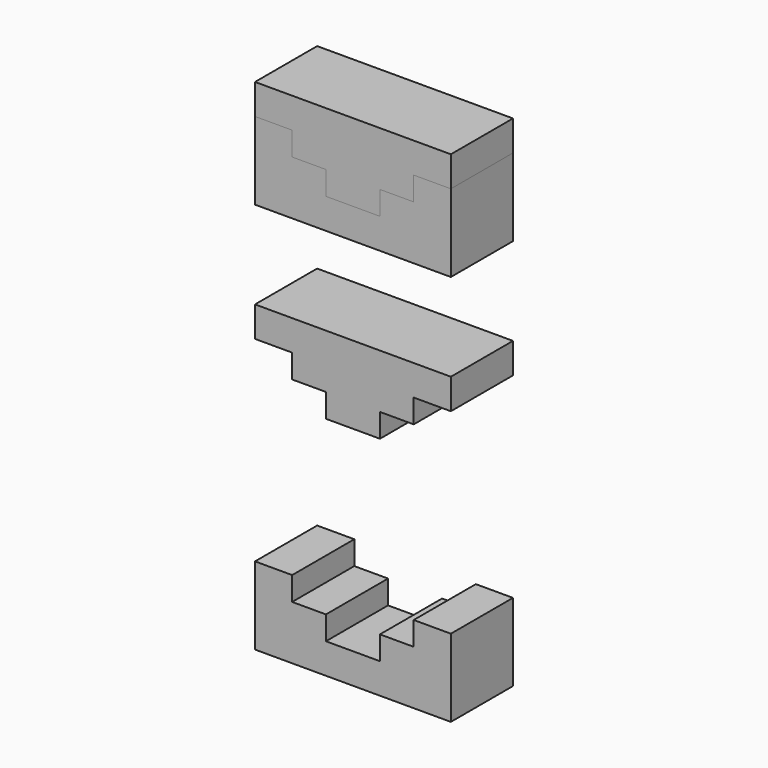
from build123d import *

# Parameters (mm, degrees)
F2_DEPTH = 23
F3_DEPTH = 23


# Not quite as in the source:
# - a feature names something its author has since deleted; it is built from what else it names


with BuildPart() as f2:
    # F1 (on Front) → F2 (new body)
    with BuildSketch(Plane.XZ):
        Polygon((30, 279), (30, 270), (41, 270), (41, 263), (51, 263), (51, 256), (59, 256), (67, 256), (67, 263), (77, 263), (77, 270), (88, 270), (88, 279), align=None)
    extrude(amount=F2_DEPTH)


with BuildPart() as f2b:
    # F1 (on Front) → F2, piece 2 (new body)
    with BuildSketch(Plane.XZ):
        Polygon((41, 212), (41, 205), (51, 205), (51, 198), (59, 198), (67, 198), (67, 205), (77, 205), (77, 212), (88, 212), (88, 221), (30, 221), (30, 212), align=None)
    extrude(amount=F2_DEPTH)


with BuildPart() as f2c:
    # F1 (on Front) → F2, piece 3 (new body)
    with BuildSketch(Plane.XZ):
        Polygon((51, 147), (41, 147), (41, 154), (30, 154), (30, 131), (88, 131), (88, 154), (77, 154), (77, 147), (67, 147), (67, 140), (59, 140), (51, 140), align=None)
    extrude(amount=F2_DEPTH)


with BuildPart() as f3:
    # F1 (on Front) → F3 (new body)
    with BuildSketch(Plane.XZ):
        Polygon((41, 270), (30, 270), (30, 247), (88, 247), (88, 270), (77, 270), (77, 263), (67, 263), (67, 256), (59, 256), (51, 256), (51, 263), (41, 263), align=None)
    extrude(amount=F3_DEPTH)


solid = Compound([f2.part, f2b.part, f2c.part, f3.part])
